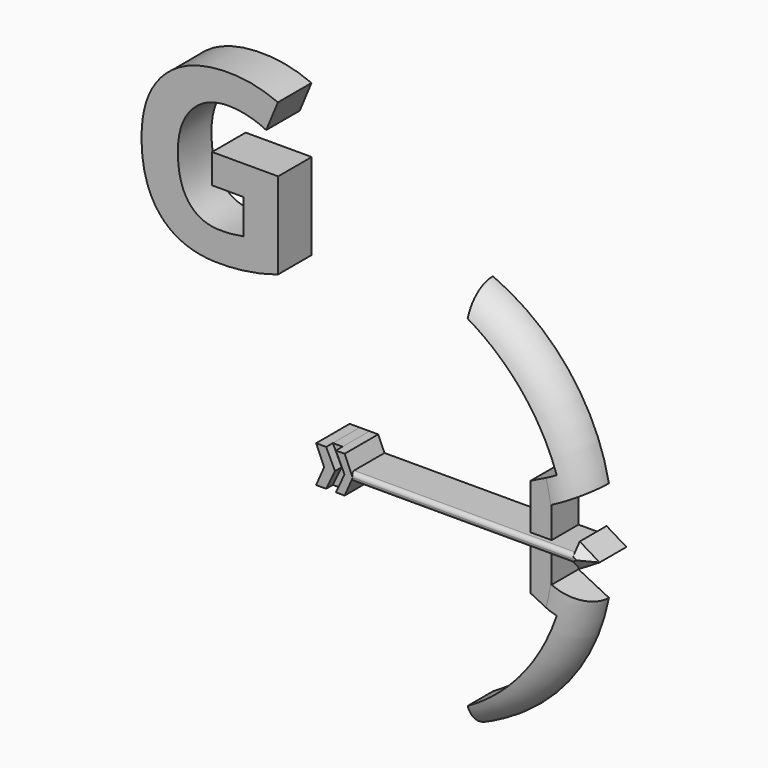
from build123d import *

# Parameters (mm, degrees)
F2_DEPTH     = 5.08
F0_TEXT_SIZE = 35.2777777778
F3_DEPTH     = 6.35
F4_R         = 0.6096
F5_R         = 5.07999
F5_2_R       = 5.07999
F6_SIZE      = 1.27


# Not quite as in the source:
# - a fillet or chamfer is up to 0.001 mm smaller than in the source, because OpenCascade refuses the exact size
# - the program builds the solid bodies; features that only make, move or delete a surface that nothing else refers to are left out
# - Text() gives the source's letters only with a copy of the font that has no kerning and outlines rounded to 1/6400 em; it was checked with that copy


with BuildPart() as f2:
    # F0 (on Front) → F2 (new body)
    with BuildSketch(Plane.XZ):
        with BuildLine():
            Line((20.290305838, 5.3244065493), (24.8951967806, 7.6268524863))
            ThreePointArc((24.8951967806, 7.6268524863), (18.8184246693, 20.7316209474), (7.339048665, 29.5000895858))
            Line((7.339048665, 29.5000895858), (7.339048665, 25.795771802))
            ThreePointArc((7.339048665, 25.795771802), (15.6297736115, 18.8312282558), (20.8659172058, 9.3536870554))
            Line((20.8659172058, 9.3536870554), (17.0680694282, 7.4645183049))
            Line((17.0680694282, 7.4645183049), (17.0680694282, 0.619783299))
            Line((17.0680694282, 0.619783299), (20.290305838, 0.619783299))
            Line((20.290305838, 0.619783299), (20.290305838, 5.3244065493))
        make_face()
    extrude(amount=F2_DEPTH)

    # F5 (radius 5.08 in the source; OpenCascade refuses exactly that, so slightly less here)
    f5_edges = [f2.edges().sort_by_distance(p)[0] for p in [
        (18.818425, -5.08, 20.731621),
    ]]
    fillet(f5_edges, radius=F5_R)


with BuildPart() as f2b:
    # F0 (on Front) → F2, piece 2 (new body)
    with BuildSketch(Plane.XZ):
        with BuildLine():
            Line((20.290305838, -5.3244065493), (20.290305838, -0.619783299))
            Line((20.290305838, -0.619783299), (17.0680694282, -0.619783299))
            Line((17.0680694282, -0.619783299), (17.0680694282, -7.4645183049))
            Line((17.0680694282, -7.4645183049), (20.8659172058, -9.3536870554))
            ThreePointArc((20.8659172058, -9.3536870554), (15.6297736115, -18.8312282558), (7.339048665, -25.795771802))
            Line((7.339048665, -25.795771802), (7.339048665, -29.5000895858))
            ThreePointArc((7.339048665, -29.5000895858), (18.8184246693, -20.7316209474), (24.8951967806, -7.6268524863))
            Line((24.8951967806, -7.6268524863), (20.290305838, -5.3244065493))
        make_face()
    extrude(amount=F2_DEPTH)

    # F5#2 (radius 5.08 in the source; OpenCascade refuses exactly that, so slightly less here)
    f5_2_edges = [f2b.edges().sort_by_distance(p)[0] for p in [
        (18.818425, -5.08, -20.731621),
    ]]
    fillet(f5_2_edges, radius=F5_2_R)


with BuildPart() as f2c:
    # F0 (on Front) → F2, piece 3 (new body)
    with BuildSketch(Plane.XZ):
        Polygon((-10.0388554856, 0), (-11.3339805976, 2.786931349), (-12.8089860082, 2.786931349), (-11.4778839052, 0), align=None)
        Polygon((-11.3339805976, -2.786931349), (-10.0388554856, 0), (-11.4778839052, 0), (-12.8089860082, -2.786931349), align=None)
    extrude(amount=F2_DEPTH)


with BuildPart() as f3:
    # F0 (on Front) → F3 (new body)
    with BuildSketch(Plane.XZ):
        Polygon((24.541143328, 0.619783299), (20.290305838, 0.619783299), (17.0680694282, 0.619783299), (-9.0640922582, 0.619783299), (-8.7925652042, 0), (-9.0640922582, -0.619783299), (17.0680694282, -0.619783299), (20.290305838, -0.619783299), (24.541143328, -0.619783299), (24.541143328, 0), align=None)
        Polygon((-11.4778839052, 0), (-12.8089860082, 2.786931349), (-14.3334493041, 2.786931349), (-13.112494722, 0), align=None)
        Polygon((-10.0135197863, 2.786931349), (-10.9029447292, 2.786931349), (-11.3339805976, 2.786931349), (-10.0388554856, 0), (-8.7925652042, 0), (-9.0640922582, 0.619783299), align=None)
        Polygon((-12.8089860082, -2.786931349), (-11.4778839052, 0), (-13.112494722, 0), (-14.3334493041, -2.786931349), align=None)
        Polygon((-8.7925652042, 0), (-10.0388554856, 0), (-11.3339805976, -2.786931349), (-10.9029447292, -2.786931349), (-10.0135197863, -2.786931349), (-9.0640922582, -0.619783299), align=None)
        with Locations((-42.7976534254, 22.3170020418)):
            Text('G', F0_TEXT_SIZE, font='Open Sans', font_style=FontStyle.BOLD, text_align=(TextAlign.LEFT, TextAlign.BOTTOM))
        Polygon((24.541143328, 1.8237228505), (24.541143328, 0.619783299), (24.541143328, 0), (24.541143328, -0.619783299), (24.541143328, -1.8237228505), (27.542905882, 0), align=None)
    extrude(amount=F3_DEPTH)

    # F4
    f4_edges = [f3.edges().sort_by_distance(p)[0] for p in [
        (7.738526, -6.35, -0.619783),
        (7.738526, -6.35, 0.619783),
    ]]
    fillet(f4_edges, radius=F4_R)

    # F6
    f6_edges = [f3.edges().sort_by_distance(p)[0] for p in [
        (26.042025, -6.35, -0.911861),
        (26.042025, -6.35, 0.911861),
    ]]
    chamfer(f6_edges, length=F6_SIZE)


solid = Compound([f2.part, f2b.part, f2c.part, f3.part])
